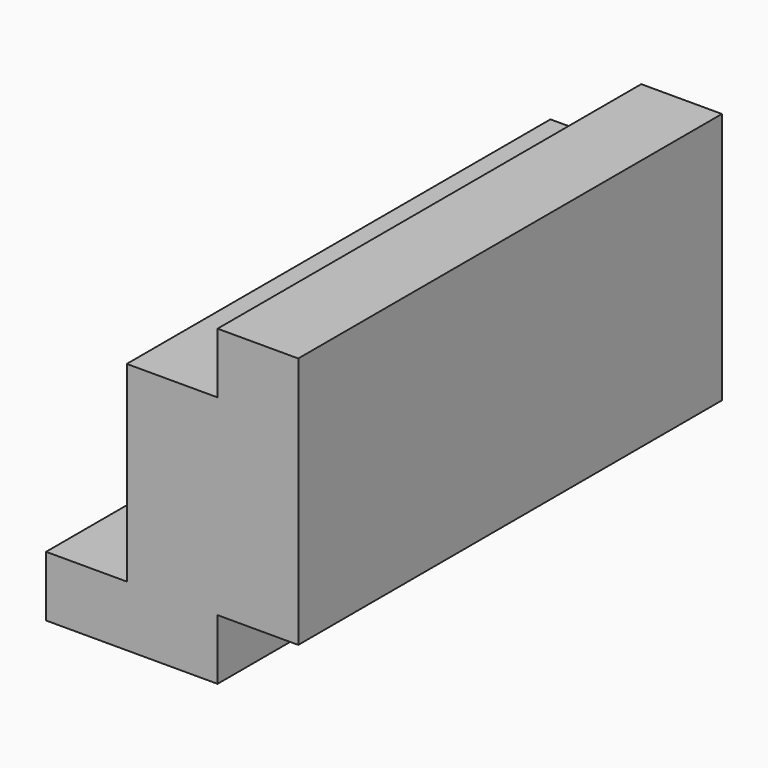
from build123d import *

# Parameters (mm, degrees)
F1_DEPTH = 105


# Not quite as in the source:
# - the program builds the solid bodies; features that only make, move or delete a surface that nothing else refers to are left out


with BuildPart() as f1:
    # F0 (on Front) → F1 (new body)
    with BuildSketch(Plane.XZ):
        Polygon((24.5621289364, 25.0425585955), (8.5621289364, 25.0425585955), (8.5621289364, 13.0425585955), (-9.4378710636, 13.0425585955), (-9.4378710636, -24.9574414045), (-25.4378710636, -24.9574414045), (-25.4378710636, -36.9574414045), (8.5621289364, -36.9574414045), (8.5621289364, -24.9574414045), (24.5621289364, -24.9574414045), align=None)
    extrude(amount=F1_DEPTH)


solid = f1.part
